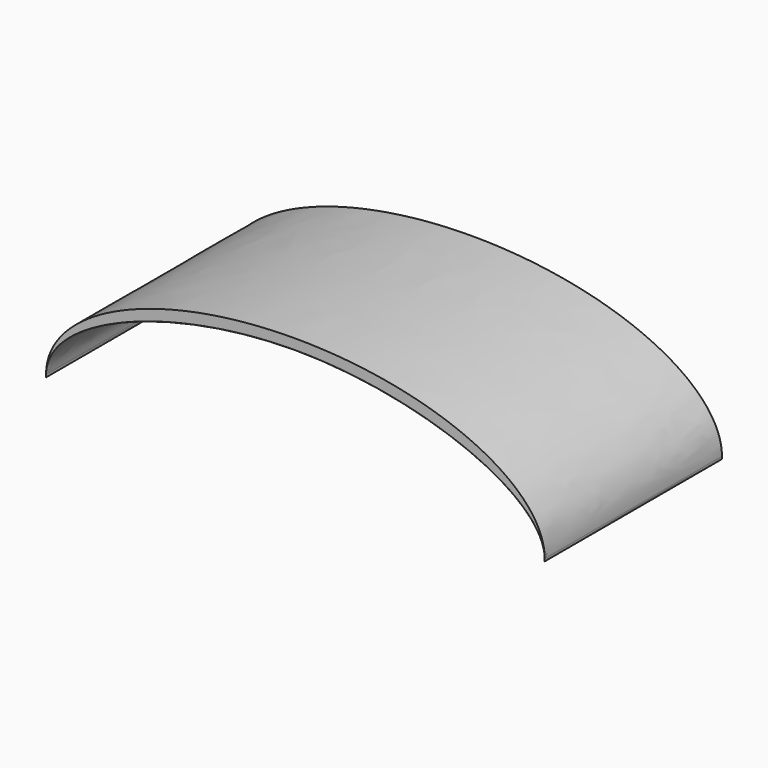
from build123d import *

# Parameters (mm, degrees)
F1_DEPTH = 50.8


with BuildPart() as f1:
    # F0 (on Front) → F1 (new body)
    with BuildSketch(Plane.XZ):
        with BuildLine():
            add(Edge.make_bspline(
                [(-57.1653934626, 0), (-57.1653934626, -0.2996959884), (-57.15, -0.5993112749)],
                knots=[3.1415926536, 3.1415926536, 3.1415926536, 3.1648000438, 3.1648000438, 3.1648000438], degree=2, weights=[1, 0.9999326779, 1]))
            add(Edge.make_bspline(
                [(-57.15, -0.5993112749), (-57.1625511192, -0.3992945688), (-57.1677226229, -0.1995037349), (-57.1653934626, 0)],
                knots=[0.9959501851, 0.9959501851, 0.9959501851, 0.9959501851, 1, 1, 1, 1], degree=3))
        make_face()
    extrude(amount=F1_DEPTH)


with BuildPart() as f1b:
    # F0 (on Front) → F1, piece 2 (new body)
    with BuildSketch(Plane.XZ):
        with BuildLine():
            add(Edge.make_bspline(
                [(57.1653934626, 0), (57.1653934626, 25.8264746088), (0, 25.8264746088), (-57.1653934626, 25.8264746088), (-57.1653934626, 0)],
                knots=[0, 0, 0, 1.5707963268, 1.5707963268, 3.1415926536, 3.1415926536, 3.1415926536], degree=2, weights=[1, 0.7071067812, 1, 0.7071067812, 1]))
            add(Edge.make_bspline(
                [(-57.1653934626, 0), (-57.0221540116, 12.2691447256), (0, 34.6357926861), (57.0221540116, 12.2691447256), (57.1653934626, 0)],
                knots=[0, 0, 0, 0, 0.2490568167, 0.4981136334, 0.4981136334, 0.4981136334, 0.4981136334], degree=3))
        make_face()
    extrude(amount=F1_DEPTH)


with BuildPart() as f1c:
    # F0 (on Front) → F1, piece 3 (new body)
    with BuildSketch(Plane.XZ):
        with BuildLine():
            add(Edge.make_bspline(
                [(57.1653934626, 0), (57.1677226229, -0.1995037349), (57.1625511192, -0.3992945688), (57.15, -0.5993112749)],
                knots=[0.4981136334, 0.4981136334, 0.4981136334, 0.4981136334, 0.5021634483, 0.5021634483, 0.5021634483, 0.5021634483], degree=3))
            add(Edge.make_bspline(
                [(57.15, -0.5993112749), (57.1653934626, -0.2996959884), (57.1653934626, 0)],
                knots=[6.2599779169, 6.2599779169, 6.2599779169, 6.2831853072, 6.2831853072, 6.2831853072], degree=2, weights=[1, 0.9999326779, 1]))
        make_face()
    extrude(amount=F1_DEPTH)


solid = Compound([f1.part, f1b.part, f1c.part])
